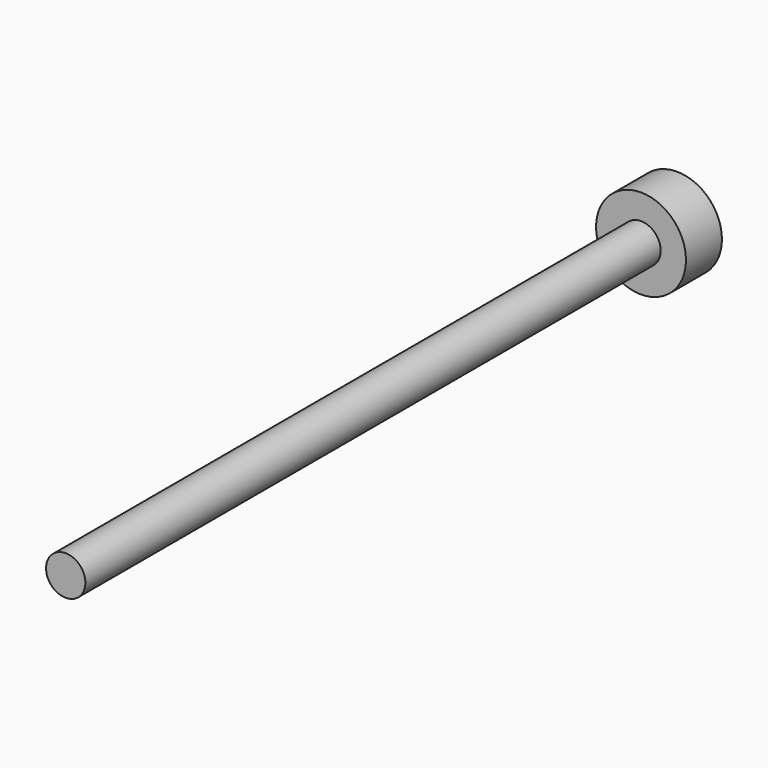
from build123d import *

# Parameters (mm, degrees)
F0_R     = 1.3890625
F1_DEPTH = 50.8
F2_R     = 3.175
F3_DEPTH = 3.175


# Not quite as in the source:
# - a feature names something its author has since deleted; it is built from what else it names


with BuildPart() as f1:
    # F0 (on Front) → F1 (new body)
    with BuildSketch(Plane.XZ):
        Circle(F0_R)
    extrude(amount=F1_DEPTH)

    # F2 (on Front) → F3 (join)
    with BuildSketch(Plane.XZ):
        Circle(F2_R)
    extrude(amount=-F3_DEPTH)


solid = f1.part
